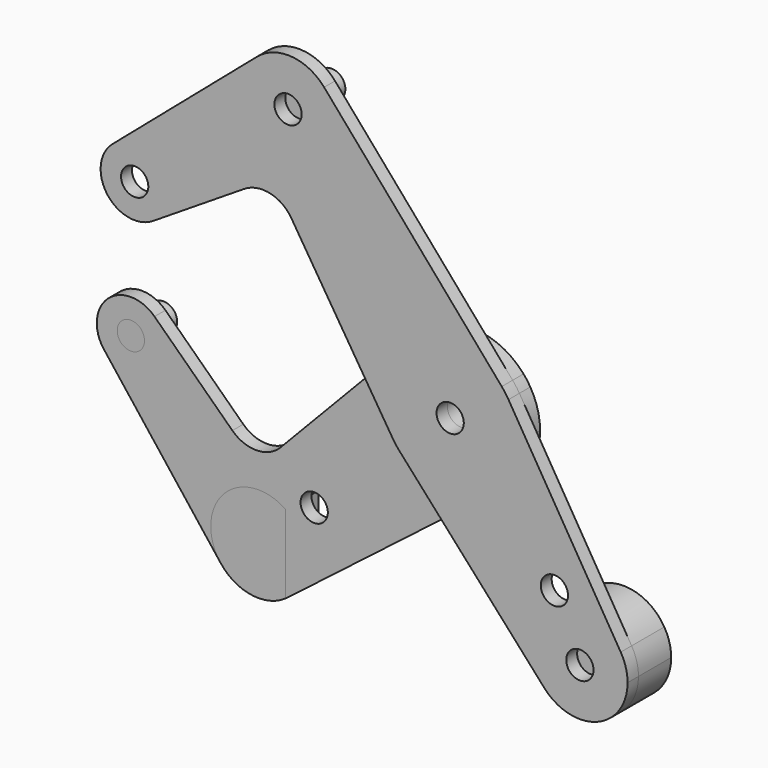
from build123d import *

# Parameters (mm, degrees)
F0_R     = 3.175
F1_DEPTH = 3.175
F2_DEPTH = 3.175
F3_DEPTH = 3.175
F6_DEPTH = 9.525
F5_R     = 3.2017905818
F7_DEPTH = 9.525


with BuildPart() as f1:
    # F0 (on Front) → F1 (new body)
    with BuildSketch(Plane.XZ):
        with BuildLine():
            ThreePointArc((9.7006393072, -12.5663527737), (14.2480397599, -7.0006419705), (15.875, 0))
            ThreePointArc((15.875, 0), (15.2928451858, 4.2596374402), (13.589077339, 8.2068631081))
            ThreePointArc((13.589077339, 8.2068631081), (12.8481306417, 9.3242245797), (12.0155447944, 10.3750811223))
            ThreePointArc((12.0155447944, 10.3750811223), (0.4046753915, 15.8698412981), (-11.4711511247, 10.9739836374))
            ThreePointArc((-11.4711511247, 10.9739836374), (-15.7947937715, 1.5937737343), (-13.4322489239, -8.461105947))
            ThreePointArc((-13.4322489239, -8.461105947), (-12.6704088261, -9.5643277432), (-11.818197177, -10.5993320773))
            ThreePointArc((-11.818197177, -10.5993320773), (-1.4450970341, -15.8090897765), (9.7006393072, -12.5663527737))
        make_face()
        Circle(F0_R, mode=Mode.SUBTRACT)
        with BuildLine():
            Line((-1.9723715397, -21.5773737034), (9.7006393072, -12.5663527737))
            ThreePointArc((9.7006393072, -12.5663527737), (-1.4450970341, -15.8090897765), (-11.818197177, -10.5993320773))
            Line((-11.818197177, -10.5993320773), (-1.9723715397, -21.5773737034))
        make_face()
        with BuildLine():
            Line((-1.9723715397, -21.5773737034), (-11.818197177, -10.5993320773))
            ThreePointArc((-11.818197177, -10.5993320773), (-12.6704088261, -9.5643277432), (-13.4322489239, -8.461105947))
            Line((-13.4322489239, -8.461105947), (-20.0354577926, 2.0216779558))
            Line((-20.0354577926, 2.0216779558), (-42.0186206254, -20.9574143581))
            ThreePointArc((-42.0186206254, -20.9574143581), (-47.601548398, -23.4101962273), (-53.2796810271, -21.1866784606))
            Line((-53.2796810271, -21.1866784606), (-71.4303764219, -3.6977333553))
            ThreePointArc((-71.4303764219, -3.6977333553), (-69.6330912018, -6.308131344), (-69.0003723469, -9.4136230398))
            ThreePointArc((-69.0003723469, -9.4136230398), (-74.3620830362, -16.921566545), (-83.2036392891, -14.2864118589))
            Line((-83.2036392891, -14.2864118589), (-55.9857223186, -49.2850811473))
            ThreePointArc((-55.9857223186, -49.2850811473), (-55.2758223722, -34.8153662876), (-40.8636484691, -33.3436837668))
            ThreePointArc((-40.8636484691, -33.3436837668), (-37.3634700126, -37.3190890389), (-36.1011484691, -42.4631769682))
            ThreePointArc((-36.1011484691, -42.4631769682), (-37.2400206372, -47.3636263476), (-40.4232009541, -51.2596239098))
            Line((-40.4232009541, -51.2596239098), (-1.9723715397, -21.5773737034))
        make_face()
        with Locations((-34.2204524104, -30.7773106666)):
            Circle(F0_R, mode=Mode.SUBTRACT)
        with BuildLine():
            ThreePointArc((-13.4322489239, -8.461105947), (-15.7947937715, 1.5937737343), (-11.4711511247, 10.9739836374))
            Line((-11.4711511247, 10.9739836374), (-20.0354577926, 2.0216779558))
            Line((-20.0354577926, 2.0216779558), (-13.4322489239, -8.461105947))
        make_face()
        with BuildLine():
            ThreePointArc((-55.9857223186, -49.2850811473), (-48.882881605, -53.4495920791), (-40.8636484691, -51.5826701696))
            Line((-40.8636484691, -51.5826701696), (-40.8636484691, -33.3436837668))
            ThreePointArc((-40.8636484691, -33.3436837668), (-55.2758223722, -34.8153662876), (-55.9857223186, -49.2850811473))
        make_face()
        with Locations((-47.2136484691, -42.4631769682)):
            Circle(F0_R, mode=Mode.SUBTRACT)
        with BuildLine():
            ThreePointArc((-71.4303764219, -3.6977333553), (-82.2457694679, -3.5119169812), (-83.2036392891, -14.2864118589))
            ThreePointArc((-83.2036392891, -14.2864118589), (-74.3620830362, -16.921566545), (-69.0003723469, -9.4136230398))
            ThreePointArc((-69.0003723469, -9.4136230398), (-69.6330912018, -6.308131344), (-71.4303764219, -3.6977333553))
        make_face()
        with Locations((-76.9378723469, -9.4136230398)):
            Circle(F0_R, mode=Mode.SUBTRACT)
    extrude(amount=-F1_DEPTH)

    # F0 (on Front) → F3 (join)
    with BuildSketch(Plane.XZ):
        with BuildLine():
            ThreePointArc((-40.8636484691, -51.5826701696), (-40.64143956, -51.4238536338), (-40.4232009541, -51.2596239098))
            ThreePointArc((-40.4232009541, -51.2596239098), (-37.2400206372, -47.3636263476), (-36.1011484691, -42.4631769682))
            ThreePointArc((-36.1011484691, -42.4631769682), (-37.3634700126, -37.3190890389), (-40.8636484691, -33.3436837668))
            Line((-40.8636484691, -33.3436837668), (-40.8636484691, -51.5826701696))
        make_face()
    extrude(amount=-F3_DEPTH)


with BuildPart() as f2:
    # F0 (on Front) → F2 (new body)
    with BuildSketch(Plane.XZ):
        with BuildLine():
            ThreePointArc((9.7006393072, -12.5663527737), (14.2480397599, -7.0006419705), (15.875, 0))
            ThreePointArc((15.875, 0), (15.2928451858, 4.2596374402), (13.589077339, 8.2068631081))
            ThreePointArc((13.589077339, 8.2068631081), (12.8481306417, 9.3242245797), (12.0155447944, 10.3750811223))
            ThreePointArc((12.0155447944, 10.3750811223), (0.4046753915, 15.8698412981), (-11.4711511247, 10.9739836374))
            ThreePointArc((-11.4711511247, 10.9739836374), (-15.7947937715, 1.5937737343), (-13.4322489239, -8.461105947))
            ThreePointArc((-13.4322489239, -8.461105947), (-12.6704088261, -9.5643277432), (-11.818197177, -10.5993320773))
            ThreePointArc((-11.818197177, -10.5993320773), (-1.4450970341, -15.8090897765), (9.7006393072, -12.5663527737))
        make_face()
        Circle(F0_R, mode=Mode.SUBTRACT)
        with BuildLine():
            ThreePointArc((13.589077339, 8.2068631081), (15.2928451858, 4.2596374402), (15.875, 0))
            ThreePointArc((15.875, 0), (14.2480397599, -7.0006419705), (9.7006393072, -12.5663527737))
            Line((9.7006393072, -12.5663527737), (-1.9723715397, -21.5773737034))
            Line((-1.9723715397, -21.5773737034), (21.9502834065, -48.2510028613))
            ThreePointArc((21.9502834065, -48.2510028613), (23.6117354925, -31.8995862557), (39.7353755677, -35.0866662316))
            Line((39.7353755677, -35.0866662316), (13.589077339, 8.2068631081))
        make_face()
        with Locations((24.2823193089, -27.4688883834)):
            Circle(F0_R, mode=Mode.SUBTRACT)
        with BuildLine():
            Line((-1.9723715397, -21.5773737034), (9.7006393072, -12.5663527737))
            ThreePointArc((9.7006393072, -12.5663527737), (-1.4450970341, -15.8090897765), (-11.818197177, -10.5993320773))
            Line((-11.818197177, -10.5993320773), (-1.9723715397, -21.5773737034))
        make_face()
        with BuildLine():
            ThreePointArc((-11.4711511247, 10.9739836374), (0.4046753915, 15.8698412981), (12.0155447944, 10.3750811223))
            Line((12.0155447944, 10.3750811223), (-29.3678954319, 58.3018947947))
            ThreePointArc((-29.3678954319, 58.3018947947), (-27.3635577476, 54.9137242302), (-26.666276788, 51.0393380091))
            ThreePointArc((-26.666276788, 51.0393380091), (-42.4219285212, 40.9433586989), (-45.0111673585, 59.4761728946))
            Line((-45.0111673585, 59.4761728946), (-78.6723066589, 30.62050489))
            ThreePointArc((-78.6723066589, 30.62050489), (-70.189776442, 31.8056080505), (-65.5688133943, 24.5941942575))
            ThreePointArc((-65.5688133943, 24.5941942575), (-66.5502150866, 20.7710276925), (-69.2517368799, 17.8932626108))
            Line((-69.2517368799, 17.8932626108), (-47.9730600876, 31.4035867439))
            ThreePointArc((-47.9730600876, 31.4035867439), (-41.9651841532, 32.4479277656), (-36.9848059896, 28.9292554649))
            Line((-36.9848059896, 28.9292554649), (-20.0354577926, 2.0216779558))
            Line((-20.0354577926, 2.0216779558), (-11.4711511247, 10.9739836374))
        make_face()
        with BuildLine():
            ThreePointArc((41.3355214304, -40.8314704072), (40.9280130605, -37.8497241991), (39.7353755677, -35.0866662316))
            ThreePointArc((39.7353755677, -35.0866662316), (23.6117354925, -31.8995862557), (21.9502834065, -48.2510028613))
            ThreePointArc((21.9502834065, -48.2510028613), (34.1952283081, -51.2097760864), (41.3355214304, -40.8314704072))
        make_face()
        with Locations((30.2230214304, -40.8314704072)):
            Circle(F0_R, mode=Mode.SUBTRACT)
        with BuildLine():
            ThreePointArc((-13.4322489239, -8.461105947), (-15.7947937715, 1.5937737343), (-11.4711511247, 10.9739836374))
            Line((-11.4711511247, 10.9739836374), (-20.0354577926, 2.0216779558))
            Line((-20.0354577926, 2.0216779558), (-13.4322489239, -8.461105947))
        make_face()
        with BuildLine():
            ThreePointArc((-26.666276788, 51.0393380091), (-27.3635577476, 54.9137242302), (-29.3678954319, 58.3018947947))
            ThreePointArc((-29.3678954319, 58.3018947947), (-36.9469460378, 62.1206607574), (-45.0111673585, 59.4761728946))
            ThreePointArc((-45.0111673585, 59.4761728946), (-42.4219285212, 40.9433586989), (-26.666276788, 51.0393380091))
        make_face()
        with Locations((-37.778776788, 51.0393380091)):
            Circle(F0_R, mode=Mode.SUBTRACT)
        with BuildLine():
            ThreePointArc((-65.5688133943, 24.5941942575), (-70.189776442, 31.8056080505), (-78.6723066589, 30.62050489))
            ThreePointArc((-78.6723066589, 30.62050489), (-79.8862306455, 19.871847159), (-69.2517368799, 17.8932626108))
            ThreePointArc((-69.2517368799, 17.8932626108), (-66.5502150866, 20.7710276925), (-65.5688133943, 24.5941942575))
        make_face()
        with Locations((-73.5063133943, 24.5941942575)):
            Circle(F0_R, mode=Mode.SUBTRACT)
    extrude(amount=F2_DEPTH)


with BuildPart() as f6:
    # F0 (on Front) → F6 (new body, through all)
    with BuildSketch(Plane.XZ):
        with BuildLine():
            ThreePointArc((41.3355214304, -40.8314704072), (40.9280130605, -37.8497241991), (39.7353755677, -35.0866662316))
            ThreePointArc((39.7353755677, -35.0866662316), (23.6117354925, -31.8995862557), (21.9502834065, -48.2510028613))
            ThreePointArc((21.9502834065, -48.2510028613), (34.1952283081, -51.2097760864), (41.3355214304, -40.8314704072))
        make_face()
        with Locations((30.2230214304, -40.8314704072)):
            Circle(F0_R, mode=Mode.SUBTRACT)
        with Locations((30.2230214304, -40.8314704072)):
            Circle(F0_R)
    extrude(amount=-F6_DEPTH)


with BuildPart() as f6b:
    # F0 (on Front) → F6, piece 2 (new body, through all)
    with BuildSketch(Plane.XZ):
        with BuildLine():
            ThreePointArc((-55.9857223186, -49.2850811473), (-48.882881605, -53.4495920791), (-40.8636484691, -51.5826701696))
            Line((-40.8636484691, -51.5826701696), (-40.8636484691, -33.3436837668))
            ThreePointArc((-40.8636484691, -33.3436837668), (-55.2758223722, -34.8153662876), (-55.9857223186, -49.2850811473))
        make_face()
        with Locations((-47.2136484691, -42.4631769682)):
            Circle(F0_R, mode=Mode.SUBTRACT)
        with Locations((-47.2136484691, -42.4631769682)):
            Circle(F0_R)
    extrude(amount=-F6_DEPTH)


with BuildPart() as f6c:
    # F5 (on Front) → F6, piece 3 (new body, through all)
    with BuildSketch(Plane.XZ):
        with Locations((-37.7789363265, 51.0394647717)):
            Circle(F5_R)
    extrude(amount=-F6_DEPTH)


with BuildPart() as f7:
    # F0 (on Front) → F7 (new body, through all)
    with BuildSketch(Plane.XZ):
        with Locations((-76.9378723469, -9.4136230398)):
            Circle(F0_R)
    extrude(amount=-F7_DEPTH)


solid = Compound([f1.part, f2.part, f6.part, f6b.part, f6c.part, f7.part])
